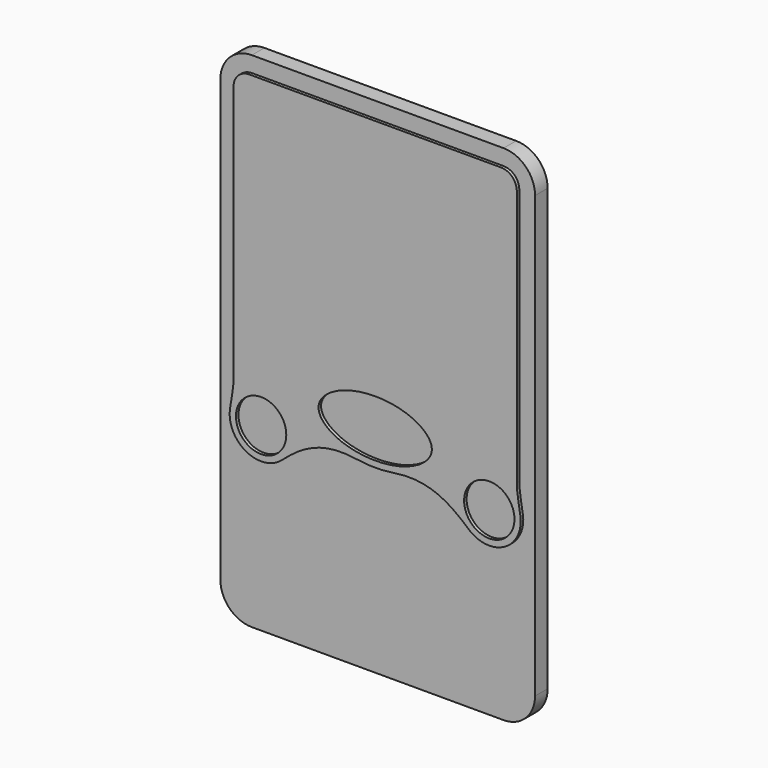
from build123d import *

# Parameters (mm, degrees)
F0_W     = 25.4
F0_H     = 40.64
F1_DEPTH = 1.27
F2_R     = 2.032
F3_DEPTH = 0.254
F4_R     = 2.54
F5_R     = 1.27


# Not quite as in the source:
# - the dataset's text gives a spline's control points without its knots; the knots are read off the source's solid


with BuildPart() as f1:
    # F0 (on Front) → F1 (new body)
    with BuildSketch(Plane.XZ):
        Rectangle(F0_W, F0_H)
    extrude(amount=F1_DEPTH)

    # F2 (on face) → F3 (join)
    with BuildSketch(Plane.XZ.offset(1.27)):
        with BuildLine():
            ThreePointArc((-7.5180080999, -7.4846331009), (-6.8898600985, -6.6273003834), (-6.6675, -5.588))
            ThreePointArc((-6.6675, -5.588), (-9.0473495717, -3.0530538782), (-11.7273045987, -5.268336451))
            ThreePointArc((-11.7273045987, -5.268336451), (-10.3908627949, -7.8354991648), (-7.5180080999, -7.4846331009))
        make_face()
        with Locations((-9.2075, -5.588)):
            Circle(F2_R, mode=Mode.SUBTRACT)
        with BuildLine():
            ThreePointArc((-11.7273045987, -5.268336451), (-9.0473495717, -3.0530538782), (-6.6675, -5.588))
            ThreePointArc((-6.6675, -5.588), (-6.8898600985, -6.6273003834), (-7.5180080999, -7.4846331009))
            add(Edge.make_bspline(
                [(-1.4182194217, -5.4769095653), (-4.1012740694, -5.0478749908), (-5.7548377663, -5.9140278026), (-7.5180080999, -7.4846331009)],
                knots=[0, 0, 0, 0, 6.4217112762, 6.4217112762, 6.4217112762, 6.4217112762], degree=3))
            add(Edge.make_bspline(
                [(-5.08, -2.794), (-5.08, -4.8913715579), (-1.4182194217, -5.4769095653)],
                knots=[3.1415926536, 3.1415926536, 3.1415926536, 4.4294520022, 4.4294520022, 4.4294520022], degree=2, weights=[1, 0.7997427872, 1]))
            add(Edge.make_bspline(
                [(5.08, -2.794), (5.08, 0), (0, 0), (-5.08, 0), (-5.08, -2.794)],
                knots=[0, 0, 0, 1.5707963268, 1.5707963268, 3.1415926536, 3.1415926536, 3.1415926536], degree=2, weights=[1, 0.7071067812, 1, 0.7071067812, 1]))
            add(Edge.make_bspline(
                [(1.4182194217, -5.4769095653), (5.08, -4.8913715579), (5.08, -2.794)],
                knots=[4.9953259586, 4.9953259586, 4.9953259586, 6.2831853072, 6.2831853072, 6.2831853072], degree=2, weights=[1, 0.7997427872, 1]))
            add(Edge.make_bspline(
                [(1.4182194217, -5.4769095653), (4.1012740694, -5.0478749908), (5.7548377663, -5.9140278026), (7.5180080999, -7.4846331009)],
                knots=[0, 0, 0, 0, 6.4217112762, 6.4217112762, 6.4217112762, 6.4217112762], degree=3))
            ThreePointArc((7.5180080999, -7.4846331009), (8.0241372051, -3.3405008352), (11.7273045987, -5.268336451))
            add(Edge.make_bspline(
                [(11.43, -2.9357403982), (11.43, -3.7171181073), (11.6289668146, -4.4931714335), (11.7273045987, -5.268336451)],
                knots=[0, 0, 0, 0, 2.3514664297, 2.3514664297, 2.3514664297, 2.3514664297], degree=3))
            Line((11.43, -2.9357403982), (11.43, 19.05))
            Line((11.43, 19.05), (-11.43, 19.05))
            Line((-11.43, 19.05), (-11.43, -2.9357403982))
            add(Edge.make_bspline(
                [(-11.43, -2.9357403982), (-11.43, -3.7171181073), (-11.6289668146, -4.4931714335), (-11.7273045987, -5.268336451)],
                knots=[0, 0, 0, 0, 2.3514664297, 2.3514664297, 2.3514664297, 2.3514664297], degree=3))
        make_face()
        with BuildLine():
            add(Edge.make_bspline(
                [(-5.08, -2.794), (-5.08, -4.8913715579), (-1.4182194217, -5.4769095653)],
                knots=[3.1415926536, 3.1415926536, 3.1415926536, 4.4294520022, 4.4294520022, 4.4294520022], degree=2, weights=[1, 0.7997427872, 1]))
            add(Edge.make_bspline(
                [(-1.4182194217, -5.4769095653), (0, -5.7036903231), (1.4182194217, -5.4769095653)],
                knots=[4.4294520022, 4.4294520022, 4.4294520022, 4.9953259586, 4.9953259586, 4.9953259586], degree=2, weights=[1, 0.960239644, 1]))
            add(Edge.make_bspline(
                [(1.4182194217, -5.4769095653), (5.08, -4.8913715579), (5.08, -2.794)],
                knots=[4.9953259586, 4.9953259586, 4.9953259586, 6.2831853072, 6.2831853072, 6.2831853072], degree=2, weights=[1, 0.7997427872, 1]))
            add(Edge.make_bspline(
                [(5.08, -2.794), (5.08, 0), (0, 0), (-5.08, 0), (-5.08, -2.794)],
                knots=[0, 0, 0, 1.5707963268, 1.5707963268, 3.1415926536, 3.1415926536, 3.1415926536], degree=2, weights=[1, 0.7071067812, 1, 0.7071067812, 1]))
        make_face()
        with BuildLine():
            add(Edge.make_bspline(
                [(-4.572, -2.794), (-4.572, -2.9169028513), (-4.5290705478, -3.1627085538), (-4.3175460933, -3.5550013791), (-3.9283471819, -3.9595979757), (-3.3716681218, -4.3337764728), (-2.6686840163, -4.6525156626), (-1.8416721788, -4.8959053951), (-0.9445084224, -5.0455757275), (0, -5.0972121363), (0.9445084224, -5.0455757275), (1.8416721788, -4.8959053951), (2.6686840163, -4.6525156626), (3.3716681218, -4.3337764728), (3.9283471819, -3.9595979757), (4.3175460933, -3.5550013791), (4.5290705478, -3.1627085538), (4.5934647261, -2.794), (4.5290705478, -2.4252914462), (4.3175460933, -2.0329986209), (3.9283471819, -1.6284020243), (3.3716681218, -1.2542235272), (2.6686840163, -0.9354843374), (1.8416721788, -0.6920946049), (0.9445084224, -0.5424242725), (0, -0.4907878637), (-0.9445084224, -0.5424242725), (-1.8416721788, -0.6920946049), (-2.6686840163, -0.9354843374), (-3.3716681218, -1.2542235272), (-3.9283471819, -1.6284020243), (-4.3175460933, -2.0329986209), (-4.5290705478, -2.4252914462), (-4.572, -2.6710971487), (-4.572, -2.794)],
                knots=[0, 0, 0, 0, 0.03125, 0.0625, 0.09375, 0.125, 0.15625, 0.1875, 0.21875, 0.25, 0.28125, 0.3125, 0.34375, 0.375, 0.40625, 0.4375, 0.46875, 0.5, 0.53125, 0.5625, 0.59375, 0.625, 0.65625, 0.6875, 0.71875, 0.75, 0.78125, 0.8125, 0.84375, 0.875, 0.90625, 0.9375, 0.96875, 1, 1, 1, 1], degree=3))
        make_face(mode=Mode.SUBTRACT)
        with BuildLine():
            ThreePointArc((11.7273045987, -5.268336451), (8.0241372051, -3.3405008352), (7.5180080999, -7.4846331009))
            ThreePointArc((7.5180080999, -7.4846331009), (10.2468003834, -7.9056399015), (11.7475, -5.588))
            ThreePointArc((11.7475, -5.588), (11.7424461218, -5.4278495717), (11.7273045987, -5.268336451))
        make_face()
        with Locations((9.2075, -5.588)):
            Circle(F2_R, mode=Mode.SUBTRACT)
    extrude(amount=F3_DEPTH)

    # F4
    f4_edges = [f1.edges().sort_by_distance(p)[0] for p in [
        (12.7, -0.635, -20.32),
        (-12.7, -0.635, -20.32),
        (-12.7, -0.635, 20.32),
        (12.7, -0.635, 20.32),
    ]]
    fillet(f4_edges, radius=F4_R)

    # F5
    f5_edges = [f1.edges().sort_by_distance(p)[0] for p in [
        (-11.43, -1.397, 19.05),
        (11.43, -1.397, 19.05),
    ]]
    fillet(f5_edges, radius=F5_R)


solid = f1.part
